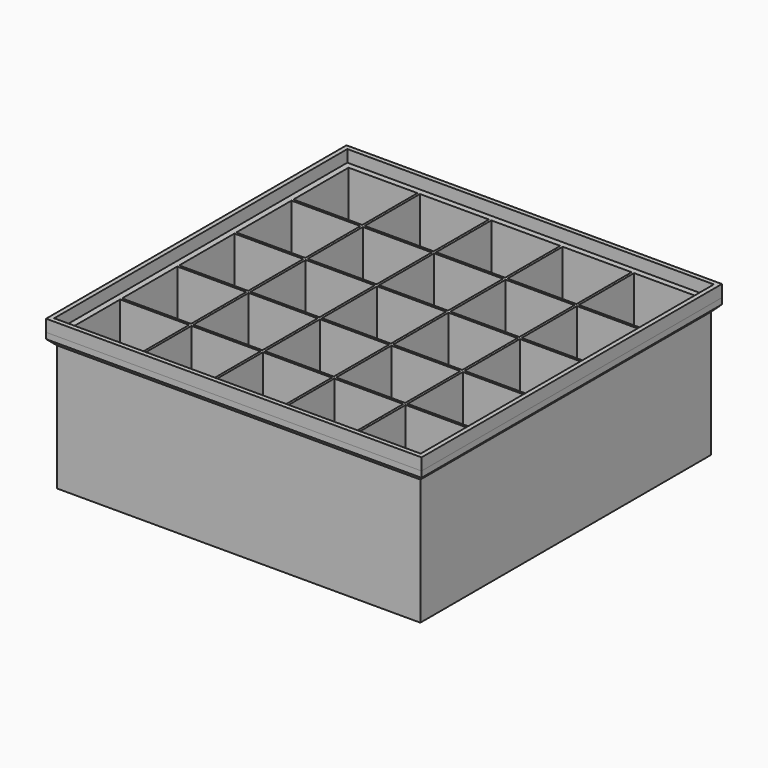
from build123d import *
from build123d import SkipClean  # not in build123d's __all__

# Parameters (mm, degrees)
F0_W      = 121.2
F0_H      = 121.2
F0_W_2    = 23
F0_H_2    = 23
F1_DEPTH  = 46
F0_R      = 8.75
F2_DEPTH  = 0.9
F3_W      = 121.2
F3_H      = 4
F4_DEPTH  = 2
F5_SIZE   = 1.99999
F7_DEPTH  = 2
F8_SIZE   = 1.99999
F9_W      = 121.2
F9_H      = 4
F10_DEPTH = 2
F11_SIZE  = 1.99999
F13_DEPTH = 2
F14_SIZE  = 1.99999
F15_W     = 1.5
F15_H     = 121.2
F16_DEPTH = 4


# Not quite as in the source:
# - a fillet or chamfer is up to 0.001 mm smaller than in the source, because OpenCascade refuses the exact size
# - a feature names something its author has since deleted; it is built from what else it names


with BuildPart() as f1:
    # F0 (on Top) → F1 (new body)
    with BuildSketch(Plane.XY):
        Rectangle(F0_W, F0_H)
        Polygon((-59.1, 35.3), (-59.1, 36.1), (-59.1, 59.1), (-36.1, 59.1), (-35.3, 59.1), (-12.3, 59.1), (-11.5, 59.1), (11.5, 59.1), (12.3, 59.1), (35.3, 59.1), (36.1, 59.1), (59.1, 59.1), (59.1, 36.1), (59.1, 35.3), (59.1, 12.3), (59.1, 11.5), (59.1, -11.5), (59.1, -12.3), (59.1, -35.3), (59.1, -36.1), (59.1, -59.1), (36.1, -59.1), (35.3, -59.1), (12.3, -59.1), (11.5, -59.1), (-11.5, -59.1), (-12.3, -59.1), (-35.3, -59.1), (-36.1, -59.1), (-59.1, -59.1), (-59.1, -36.1), (-59.1, -35.3), (-59.1, -12.3), (-59.1, -11.5), (-59.1, 11.5), (-59.1, 12.3), align=None, mode=Mode.SUBTRACT)
        Polygon((-36.1, 36.1), (-59.1, 36.1), (-59.1, 35.3), (-36.1, 35.3), (-36.1, 12.3), (-59.1, 12.3), (-59.1, 11.5), (-36.1, 11.5), (-36.1, -11.5), (-59.1, -11.5), (-59.1, -12.3), (-36.1, -12.3), (-36.1, -35.3), (-59.1, -35.3), (-59.1, -36.1), (-36.1, -36.1), (-36.1, -59.1), (-35.3, -59.1), (-35.3, -36.1), (-12.3, -36.1), (-12.3, -59.1), (-11.5, -59.1), (-11.5, -36.1), (11.5, -36.1), (11.5, -59.1), (12.3, -59.1), (12.3, -36.1), (35.3, -36.1), (35.3, -59.1), (36.1, -59.1), (36.1, -36.1), (59.1, -36.1), (59.1, -35.3), (36.1, -35.3), (36.1, -12.3), (59.1, -12.3), (59.1, -11.5), (36.1, -11.5), (36.1, 11.5), (59.1, 11.5), (59.1, 12.3), (36.1, 12.3), (36.1, 35.3), (59.1, 35.3), (59.1, 36.1), (36.1, 36.1), (36.1, 59.1), (35.3, 59.1), (35.3, 36.1), (12.3, 36.1), (12.3, 59.1), (11.5, 59.1), (11.5, 36.1), (-11.5, 36.1), (-11.5, 59.1), (-12.3, 59.1), (-12.3, 36.1), (-35.3, 36.1), (-35.3, 59.1), (-36.1, 59.1), align=None)
        with Locations((-23.8, -23.8)):
            Rectangle(F0_W_2, F0_H_2, mode=Mode.SUBTRACT)
        with Locations((0, -23.8)):
            Rectangle(F0_W_2, F0_H_2, mode=Mode.SUBTRACT)
        with Locations((-23.8, 0)):
            Rectangle(F0_W_2, F0_H_2, mode=Mode.SUBTRACT)
        Rectangle(F0_W_2, F0_H_2, mode=Mode.SUBTRACT)
        with Locations((23.8, -23.8)):
            Rectangle(F0_W_2, F0_H_2, mode=Mode.SUBTRACT)
        with Locations((23.8, 0)):
            Rectangle(F0_W_2, F0_H_2, mode=Mode.SUBTRACT)
        with Locations((-23.8, 23.8)):
            Rectangle(F0_W_2, F0_H_2, mode=Mode.SUBTRACT)
        with Locations((0, 23.8)):
            Rectangle(F0_W_2, F0_H_2, mode=Mode.SUBTRACT)
        with Locations((23.8, 23.8)):
            Rectangle(F0_W_2, F0_H_2, mode=Mode.SUBTRACT)
    extrude(amount=F1_DEPTH)

    # F0 (on Top) → F2 (join)
    with BuildSketch(Plane.XY):
        with Locations((-47.6, 47.6)):
            Rectangle(F0_W_2, F0_H_2)
        with Locations((-47.6, 47.6)):
            Circle(F0_R, mode=Mode.SUBTRACT)
        with Locations((-23.8, 47.6)):
            Rectangle(F0_W_2, F0_H_2)
        with Locations((-23.8, 47.6)):
            Circle(F0_R, mode=Mode.SUBTRACT)
        with Locations((0, 47.6)):
            Rectangle(F0_W_2, F0_H_2)
        with Locations((0, 47.6)):
            Circle(F0_R, mode=Mode.SUBTRACT)
        with Locations((23.8, 47.6)):
            Rectangle(F0_W_2, F0_H_2)
        with Locations((23.8, 47.6)):
            Circle(F0_R, mode=Mode.SUBTRACT)
        with Locations((47.6, 47.6)):
            Rectangle(F0_W_2, F0_H_2)
        with Locations((47.6, 47.6)):
            Circle(F0_R, mode=Mode.SUBTRACT)
        with Locations((47.6, 23.8)):
            Rectangle(F0_W_2, F0_H_2)
        with Locations((47.6, 23.8)):
            Circle(F0_R, mode=Mode.SUBTRACT)
        with Locations((23.8, 23.8)):
            Rectangle(F0_W_2, F0_H_2)
        with Locations((23.8, 23.8)):
            Circle(F0_R, mode=Mode.SUBTRACT)
        with Locations((0, 23.8)):
            Rectangle(F0_W_2, F0_H_2)
        with Locations((0, 23.8)):
            Circle(F0_R, mode=Mode.SUBTRACT)
        with Locations((-23.8, 23.8)):
            Rectangle(F0_W_2, F0_H_2)
        with Locations((-23.8, 23.8)):
            Circle(F0_R, mode=Mode.SUBTRACT)
        with Locations((-47.6, 23.8)):
            Rectangle(F0_W_2, F0_H_2)
        with Locations((-47.6, 23.8)):
            Circle(F0_R, mode=Mode.SUBTRACT)
        with Locations((-47.6, 0)):
            Rectangle(F0_W_2, F0_H_2)
        with Locations((-47.6, 0)):
            Circle(F0_R, mode=Mode.SUBTRACT)
        with Locations((-23.8, 0)):
            Rectangle(F0_W_2, F0_H_2)
        with Locations((-23.8, 0)):
            Circle(F0_R, mode=Mode.SUBTRACT)
        Rectangle(F0_W_2, F0_H_2)
        Circle(F0_R, mode=Mode.SUBTRACT)
        with Locations((23.8, 0)):
            Rectangle(F0_W_2, F0_H_2)
        with Locations((23.8, 0)):
            Circle(F0_R, mode=Mode.SUBTRACT)
        with Locations((47.6, 0)):
            Rectangle(F0_W_2, F0_H_2)
        with Locations((47.6, 0)):
            Circle(F0_R, mode=Mode.SUBTRACT)
        with Locations((47.6, -23.8)):
            Rectangle(F0_W_2, F0_H_2)
        with Locations((47.6, -23.8)):
            Circle(F0_R, mode=Mode.SUBTRACT)
        with Locations((23.8, -23.8)):
            Rectangle(F0_W_2, F0_H_2)
        with Locations((23.8, -23.8)):
            Circle(F0_R, mode=Mode.SUBTRACT)
        with Locations((0, -23.8)):
            Rectangle(F0_W_2, F0_H_2)
        with Locations((0, -23.8)):
            Circle(F0_R, mode=Mode.SUBTRACT)
        with Locations((-23.8, -23.8)):
            Rectangle(F0_W_2, F0_H_2)
        with Locations((-23.8, -23.8)):
            Circle(F0_R, mode=Mode.SUBTRACT)
        with Locations((-47.6, -23.8)):
            Rectangle(F0_W_2, F0_H_2)
        with Locations((-47.6, -23.8)):
            Circle(F0_R, mode=Mode.SUBTRACT)
        with Locations((-47.6, -47.6)):
            Rectangle(F0_W_2, F0_H_2)
        with Locations((-47.6, -47.6)):
            Circle(F0_R, mode=Mode.SUBTRACT)
        with Locations((-23.8, -47.6)):
            Rectangle(F0_W_2, F0_H_2)
        with Locations((-23.8, -47.6)):
            Circle(F0_R, mode=Mode.SUBTRACT)
        with Locations((0, -47.6)):
            Rectangle(F0_W_2, F0_H_2)
        with Locations((0, -47.6)):
            Circle(F0_R, mode=Mode.SUBTRACT)
        with Locations((23.8, -47.6)):
            Rectangle(F0_W_2, F0_H_2)
        with Locations((23.8, -47.6)):
            Circle(F0_R, mode=Mode.SUBTRACT)
        with Locations((47.6, -47.6)):
            Rectangle(F0_W_2, F0_H_2)
        with Locations((47.6, -47.6)):
            Circle(F0_R, mode=Mode.SUBTRACT)
    extrude(amount=F2_DEPTH)

    # F3 (on face) → F4 (join)
    with BuildSketch(Plane(origin=(-60.6, 0, 0), x_dir=(0, -1, 0), z_dir=(-1, 0, 0))):
        with Locations((0, 44)):
            Rectangle(F3_W, F3_H)
    extrude(amount=F4_DEPTH)

    # F5 (size 2 in the source; OpenCascade refuses exactly that, so slightly less here)
    f5_edges = [f1.edges().sort_by_distance(p)[0] for p in [
        (-62.6, 0, 42),
    ]]
    chamfer(f5_edges, length=F5_SIZE)

    # F6 (on face) → F7 (join)
    with BuildSketch(Plane.XZ.offset(60.6)):
        Polygon((-62.6, 44), (-60.6, 42), (60.6, 42), (60.6, 46), (-62.6, 46), align=None)
    with SkipClean():  # cleaning this boolean's faces spoils the solid; the shape is the same uncleaned
        extrude(amount=F7_DEPTH)

    # F8 (size 2 in the source; OpenCascade refuses exactly that, so slightly less here)
    f8_edges = [f1.edges().sort_by_distance(p)[0] for p in [
        (0, -62.6, 42),
    ]]
    chamfer(f8_edges, length=F8_SIZE)

    # F9 (on face) → F10 (join)
    with BuildSketch(Plane.YZ.offset(60.6)):
        with Locations((0, 44)):
            Rectangle(F9_W, F9_H)
        Polygon((-60.6, 42), (-60.6, 46), (-62.6, 46), (-62.6, 44), align=None)
    with SkipClean():  # cleaning this boolean's faces spoils the solid; the shape is the same uncleaned
        extrude(amount=F10_DEPTH)

    # F11 (size 2 in the source; OpenCascade refuses exactly that, so slightly less here)
    f11_edges = [f1.edges().sort_by_distance(p)[0] for p in [
        (62.6, 0, 42),
    ]]
    chamfer(f11_edges, length=F11_SIZE)

    # F12 (on face) → F13 (join)
    with BuildSketch(Plane(origin=(0, 60.6, 0), x_dir=(-1, 0, 0), z_dir=(0, 1, 0))):
        Polygon((62.6, 44), (62.6, 46), (-60.6, 46), (-60.6, 42), (60.6, 42), align=None)
        Polygon((-60.6, 42), (-60.6, 46), (-62.6, 46), (-62.6, 44), align=None)
    with SkipClean():  # cleaning this boolean's faces spoils the solid; the shape is the same uncleaned
        extrude(amount=F13_DEPTH)

    # F14 (size 2 in the source; OpenCascade refuses exactly that, so slightly less here)
    f14_edges = [f1.edges().sort_by_distance(p)[0] for p in [
        (0, 62.6, 42),
    ]]
    chamfer(f14_edges, length=F14_SIZE)

    # F15 (on face) → F16 (join)
    with BuildSketch(Plane.XY.offset(46)):
        Polygon((62.6, 62.6), (-62.6, 62.6), (-62.6, 60.6), (-61.1, 60.6), (-61.1, 61.1), (61.1, 61.1), (61.1, 60.6), (62.6, 60.6), align=None)
        with Locations((-61.85, 0)):
            Rectangle(F15_W, F15_H)
        Polygon((-61.1, -60.6), (-62.6, -60.6), (-62.6, -62.6), (60.6, -62.6), (60.6, -61.1), (-61.1, -61.1), align=None)
        Polygon((62.6, -62.6), (62.6, 60.6), (61.1, 60.6), (61.1, -61.1), (60.6, -61.1), (60.6, -62.6), align=None)
    with SkipClean():  # cleaning this boolean's faces spoils the solid; the shape is the same uncleaned
        extrude(amount=F16_DEPTH)


solid = f1.part
